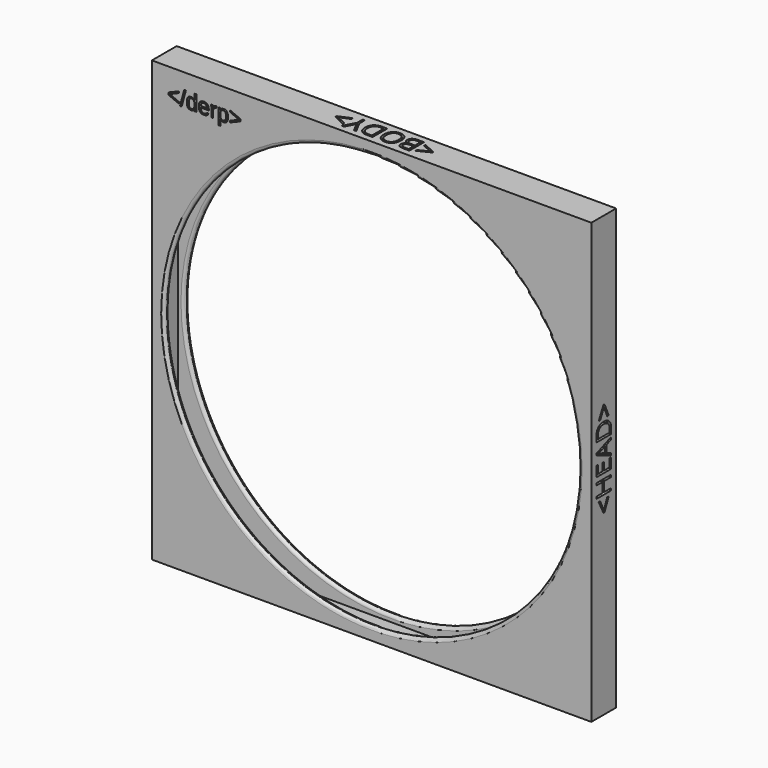
from build123d import *

# Parameters (mm, degrees)
F0_W          = 71
F0_H          = 71
F0_R          = 33.5
F1_DEPTH      = 5
F4_T          = -1
F5_R          = 0.49999
F6_R          = 3
F7_DEPTH      = 5
F2_TEXT_SIZE  = 3.4722222222
F8_DEPTH      = 0.5
F3_TEXT_SIZE  = 4.1666666667
F9_DEPTH      = 0.5
F10_TEXT_SIZE = 4.1666666667
F11_DEPTH     = 0.5
F12_TEXT_SIZE = 4.1666666667
F13_DEPTH     = 0.5
F14_TEXT_SIZE = 4.1666666667
F15_DEPTH     = 0.5


# Not quite as in the source:
# - a fillet or chamfer is up to 0.001 mm smaller than in the source, because OpenCascade refuses the exact size
# - Text() gives the source's letters only with a copy of the font that has no kerning and outlines rounded to 1/6400 em; it was checked with that copy


with BuildPart() as f1:
    # F0 (on Front) → F1 (new body)
    with BuildSketch(Plane.XZ):
        Rectangle(F0_W, F0_H)
        Circle(F0_R, mode=Mode.SUBTRACT)
    extrude(amount=F1_DEPTH)

    # F4
    f4_openings = [f1.faces().sort_by_distance(p)[0] for p in [
        (-33.5, -2.5, 0),
    ]]
    offset(amount=F4_T, openings=f4_openings)

    # F5 (radius 0.5 in the source; OpenCascade refuses exactly that, so slightly less here)
    f5_edges = [f1.edges().sort_by_distance(p)[0] for p in [
        (-33.5, -5, 0),
        (-33.5, -4, 0),
        (-33.5, -1, 0),
        (-33.5, 0, 0),
    ]]
    fillet(f5_edges, radius=F5_R)

    # F6 (on Front) → F7 (join, through all)
    with BuildSketch(Plane.XZ):
        with Locations((-29.5, -29.5)):
            Circle(F6_R)
        with Locations((-29.5, 29.5)):
            Circle(F6_R)
        with Locations((29.5, -29.5)):
            Circle(F6_R)
        with Locations((29.5, 29.5)):
            Circle(F6_R)
    extrude(amount=F7_DEPTH)

    # F2 (on face) → F8 (cut)
    with BuildSketch(Plane.XZ.offset(5)):
        with Locations((-33, 30.5)):
            Text('</derp>', F2_TEXT_SIZE, font='Arimo', text_align=(TextAlign.LEFT, TextAlign.BOTTOM))
    extrude(amount=-F8_DEPTH, mode=Mode.SUBTRACT)

    # F3 (on face) → F9 (cut)
    with BuildSketch(Plane(origin=(0, 0, -35.5), x_dir=(1, 0, 0), z_dir=(0, 0, -1))):
        with Locations((-8.1642656848, 1)):
            Text('<HTML>', F3_TEXT_SIZE, font='Open Sans', text_align=(TextAlign.LEFT, TextAlign.BOTTOM))
    extrude(amount=-F9_DEPTH, mode=Mode.SUBTRACT)

    # F10 (on face) → F11 (cut)
    with BuildSketch(Plane.YZ.offset(35.5)):
        with Locations(Location((-1, -7), (0, 0, 90))):
            Text('<HEAD>', F10_TEXT_SIZE, font='Open Sans', text_align=(TextAlign.LEFT, TextAlign.BOTTOM))
    extrude(amount=-F11_DEPTH, mode=Mode.SUBTRACT)

    # F12 (on face) → F13 (cut)
    with BuildSketch(Plane.XY.offset(35.5)):
        with Locations(Location((8.0675, -1), (0, 0, 180))):
            Text('<BODY>', F12_TEXT_SIZE, font='Open Sans', text_align=(TextAlign.LEFT, TextAlign.BOTTOM))
    extrude(amount=-F13_DEPTH, mode=Mode.SUBTRACT)

    # F14 (on face) → F15 (cut)
    with BuildSketch(Plane(origin=(-35.5, 0, 0), x_dir=(0, -1, 0), z_dir=(-1, 0, 0))):
        with Locations(Location((1, 7.2532526624), (0, 0, -90))):
            Text('<TITLE>', F14_TEXT_SIZE, font='Open Sans', text_align=(TextAlign.LEFT, TextAlign.BOTTOM))
    extrude(amount=-F15_DEPTH, mode=Mode.SUBTRACT)


solid = f1.part
